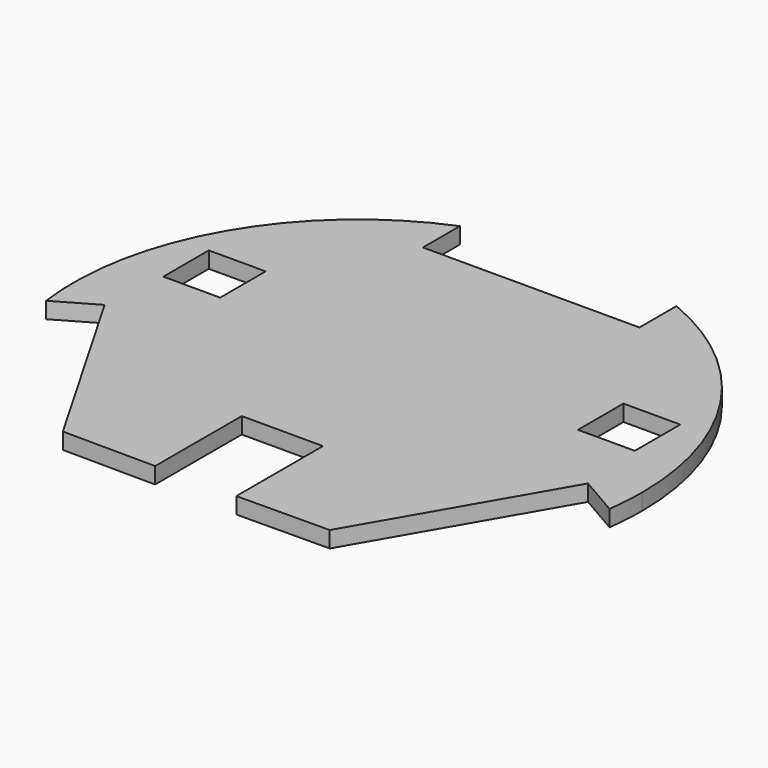
from build123d import *

# Parameters (mm, degrees)
F1_DEPTH = 6
F3_DEPTH = 25


# Not quite as in the source:
# - a feature names something its author has since deleted; it is built from what else it names


with BuildPart() as f1:
    # F0 (on Top) → F1 (new body)
    with BuildSketch(Plane.XY):
        with BuildLine():
            ThreePointArc((104.075858604, -13.900203446), (104.7687099124, -6.9654449456), (105, 0))
            ThreePointArc((105, 0), (87.2496418331, 58.4166072277), (40, 97.0824391947))
            Line((40, 97.0824391947), (40, 80))
            Line((40, 80), (0, 80))
            Line((0, 80), (-40, 80))
            Line((-40, 80), (-40, 97.0824391947))
            ThreePointArc((-40, 97.0824391947), (-90.9326673974, 52.5), (-104.075858604, -13.900203446))
            Line((-104.075858604, -13.900203446), (-89.2820323028, -5.3589838486))
            Line((-89.2820323028, -5.3589838486), (-95.2820323028, 5.0333209968))
            Line((-95.2820323028, 5.0333209968), (-71.0910346562, 19))
            Line((-71.0910346562, 19), (-87.0824391947, 19))
            Line((-87.0824391947, 19), (-87.0824391947, 40))
            Line((-87.0824391947, 40), (-66.0824391947, 40))
            Line((-66.0824391947, 40), (-66.0824391947, 21.8917139379))
            Line((-66.0824391947, 21.8917139379), (-56.3108891325, 27.5333209968))
            Line((-56.3108891325, 27.5333209968), (-30.3108891325, -17.5))
            Line((-30.3108891325, -17.5), (-30.3108891325, 35))
            Line((-30.3108891325, 35), (30.3108891325, 35))
            Line((30.3108891325, 35), (30.3108891325, -17.5))
            Line((30.3108891325, -17.5), (56.3108891325, 27.5333209968))
            Line((56.3108891325, 27.5333209968), (66.0824391947, 21.8917139379))
            Line((66.0824391947, 21.8917139379), (66.0824391947, 40))
            Line((66.0824391947, 40), (87.0824391947, 40))
            Line((87.0824391947, 40), (87.0824391947, 19))
            Line((87.0824391947, 19), (71.0910346562, 19))
            Line((71.0910346562, 19), (95.2820323028, 5.0333209968))
            Line((95.2820323028, 5.0333209968), (89.2820323028, -5.3589838486))
            Line((89.2820323028, -5.3589838486), (104.075858604, -13.900203446))
        make_face()
        Polygon((-95.2820323028, 5.0333209968), (-89.2820323028, -5.3589838486), (-69.2820323028, -40), (-30.3108891325, -17.5), (-56.3108891325, 27.5333209968), (-66.0824391947, 21.8917139379), (-66.0824391947, 19), (-71.0910346562, 19), align=None)
        Polygon((0, -17.5), (30.3108891325, -17.5), (30.3108891325, 35), (-30.3108891325, 35), (-30.3108891325, -17.5), align=None)
        Polygon((69.2820323028, -40), (89.2820323028, -5.3589838486), (95.2820323028, 5.0333209968), (71.0910346562, 19), (66.0824391947, 19), (66.0824391947, 21.8917139379), (56.3108891325, 27.5333209968), (30.3108891325, -17.5), align=None)
        Polygon((-49.2820323028, -74.6410161514), (0, -75), (0, -17.5), (-30.3108891325, -17.5), (-69.2820323028, -40), align=None)
        Polygon((0, -75), (49.2820323028, -74.6410161514), (69.2820323028, -40), (30.3108891325, -17.5), (0, -17.5), align=None)
    extrude(amount=F1_DEPTH)

    # F2 (on face) → F3 (cut)
    with BuildSketch(Plane.XY.offset(6)):
        Polygon((-14.9996020609, -74.890738782), (0, -75), (14.9996020609, -74.890738782), (15.0003979391, -34.890738782), (-14.9996020609, -34.890738782), align=None)
    extrude(amount=-F3_DEPTH, mode=Mode.SUBTRACT)


solid = f1.part
